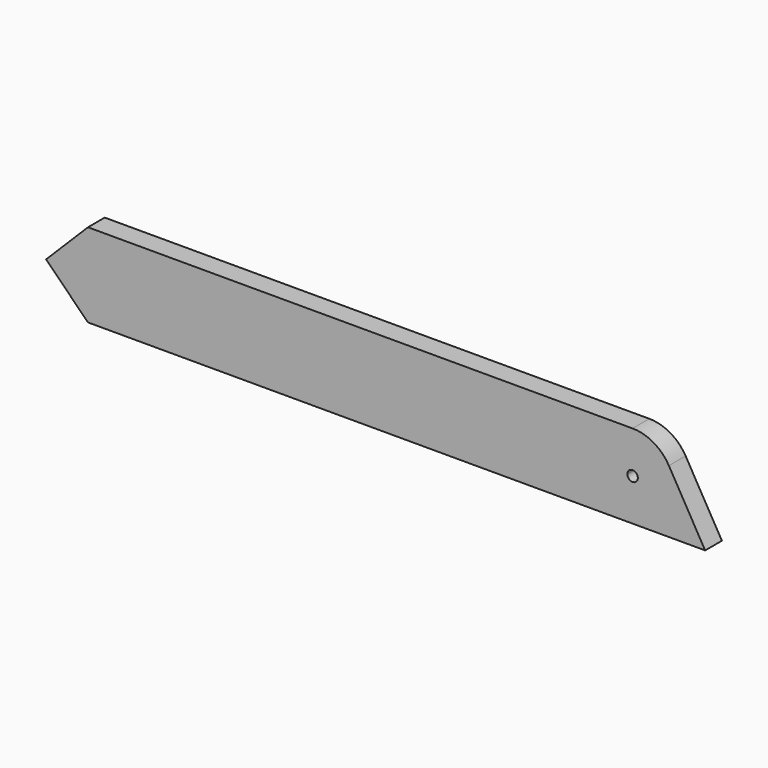
from build123d import *

# Parameters (mm, degrees)
F1_DEPTH = 3.175


with BuildPart() as f1:
    # F0 (on Front) → F1 (new body, symmetric)
    with BuildSketch(Plane.XZ):
        Polygon((65.991136, -139.7), (-77.111819, -139.7), (-77.111819, -152.4), (73.323484, -152.4), align=None)
        Polygon((-77.111819, -152.4), (-89.811819, -152.4), (-77.111819, -165.1), align=None)
        Polygon((-77.111819, -139.7), (-89.811819, -152.4), (-77.111819, -152.4), align=None)
        with BuildLine():
            Line((-77.111819, -152.4), (-77.111819, -165.1))
            Line((-77.111819, -165.1), (87.988181, -165.1))
            ThreePointArc((87.988181, -165.1), (81.638181, -163.398523), (76.989658, -158.75))
            Line((76.989658, -158.75), (73.323484, -152.4))
            Line((73.323484, -152.4), (-77.111819, -152.4))
        make_face()
        with BuildLine():
            Line((80.655833, -139.7), (65.991136, -139.7))
            Line((65.991136, -139.7), (73.323484, -152.4))
            Line((73.323484, -152.4), (75.288181, -152.4))
            ThreePointArc((75.288181, -152.4), (76.989658, -146.05), (81.638181, -141.401477))
            Line((81.638181, -141.401477), (80.655833, -139.7))
        make_face()
        with BuildLine():
            Line((75.288181, -152.4), (73.323484, -152.4))
            Line((73.323484, -152.4), (76.989658, -158.75))
            ThreePointArc((76.989658, -158.75), (75.720923, -155.687002), (75.288181, -152.4))
        make_face()
        with BuildLine():
            ThreePointArc((76.989658, -158.75), (81.638181, -163.398523), (87.988181, -165.1))
            ThreePointArc((87.988181, -165.1), (96.968437, -161.380256), (100.688181, -152.4))
            ThreePointArc((100.688181, -152.4), (100.255439, -149.112998), (98.986704, -146.05))
            ThreePointArc((98.986704, -146.05), (94.338181, -141.401477), (87.988181, -139.7))
            ThreePointArc((87.988181, -139.7), (84.701179, -140.132742), (81.638181, -141.401477))
            Line((81.638181, -141.401477), (87.194431, -151.025185))
            ThreePointArc((87.194431, -151.025185), (88.781931, -151.025185), (89.575681, -152.4))
            ThreePointArc((89.575681, -152.4), (87.988181, -153.9875), (86.400681, -152.4))
            Line((86.400681, -152.4), (75.288181, -152.4))
            ThreePointArc((75.288181, -152.4), (75.720923, -155.687002), (76.989658, -158.75))
        make_face()
        with BuildLine():
            ThreePointArc((81.638181, -141.401477), (76.989658, -146.05), (75.288181, -152.4))
            Line((75.288181, -152.4), (86.400681, -152.4))
            ThreePointArc((86.400681, -152.4), (86.613366, -151.60625), (87.194431, -151.025185))
            Line((87.194431, -151.025185), (81.638181, -141.401477))
        make_face()
        with BuildLine():
            Line((87.988181, -139.7), (80.655833, -139.7))
            Line((80.655833, -139.7), (81.638181, -141.401477))
            ThreePointArc((81.638181, -141.401477), (84.701179, -140.132742), (87.988181, -139.7))
        make_face()
        with BuildLine():
            ThreePointArc((100.688181, -152.4), (96.968437, -161.380256), (87.988181, -165.1))
            Line((87.988181, -165.1), (109.985226, -165.1))
            Line((109.985226, -165.1), (98.986704, -146.05))
            ThreePointArc((98.986704, -146.05), (100.255439, -149.112998), (100.688181, -152.4))
        make_face()
    extrude(amount=F1_DEPTH, both=True)


solid = f1.part
